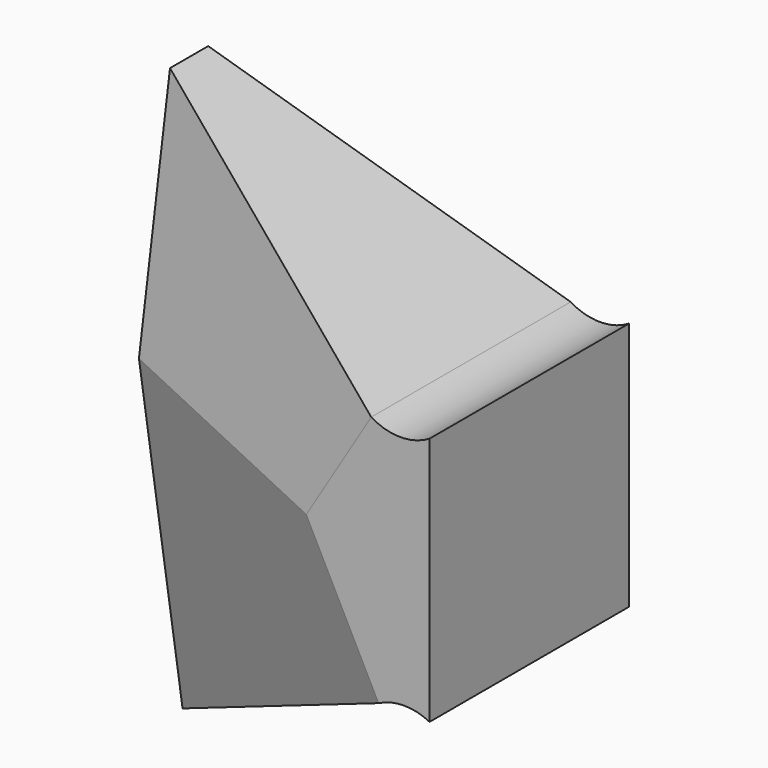
from build123d import *

# Parameters (mm, degrees)
F1_DEPTH = 38.1
F3_DEPTH = 101.6
F5_DEPTH = 127


with BuildPart() as f1:
    # F0 (on Front) → F1 (new body)
    with BuildSketch(Plane.XZ):
        with BuildLine():
            Line((27.7732536197, -17.7548748881), (27.7732536197, 20.3451251119))
            ThreePointArc((27.7732536197, 20.3451251119), (23.3150850981, 19.0968449339), (18.8569165766, 20.3451251119))
            Line((18.8569165766, 20.3451251119), (-24.5568101805, 46.7248205056))
            Line((-24.5568101805, 46.7248205056), (-24.5568101805, -40.3753659966))
            Line((-24.5568101805, -40.3753659966), (20.0085155666, -17.7548748881))
            ThreePointArc((20.0085155666, -17.7548748881), (23.8908845931, -16.8259725337), (27.7732536197, -17.7548748881))
        make_face()
    extrude(amount=F1_DEPTH)

    # F2 (on face) → F3 (cut)
    with BuildSketch(Plane(origin=(11.2647537366, 0, -22.1930380433), x_dir=(0.8917070033, 0, 0.4526131022), z_dir=(0.4526131022, 0, -0.8917070033))):
        Polygon((-40.1718992738, 0), (9.8056444527, 0), (-40.1718992738, 17.5163969398), align=None)
        Polygon((-40.1718992738, 19.8567565531), (9.8056444527, 38.1), (-40.1718992738, 38.1), align=None)
    extrude(amount=-F3_DEPTH, mode=Mode.SUBTRACT)

    # F4 (on face) → F5 (cut)
    with BuildSketch(Plane(origin=(14.113699436, 0, 23.2272693714), x_dir=(0.8546009204, 0, -0.5192853424), z_dir=(0.5192853424, 0, 0.8546009204))):
        Polygon((-25.222287783, -38.1), (5.5502130028, -38.1), (-45.2497869972, -22.2575453606), (-45.2497869972, -34.247172677), align=None)
        Polygon((-45.2497869972, -14.9671534034), (5.5502130028, 0), (-25.222287783, 0), (-45.2497869972, -3.6993231454), align=None)
    extrude(amount=-F5_DEPTH, mode=Mode.SUBTRACT)


solid = f1.part
